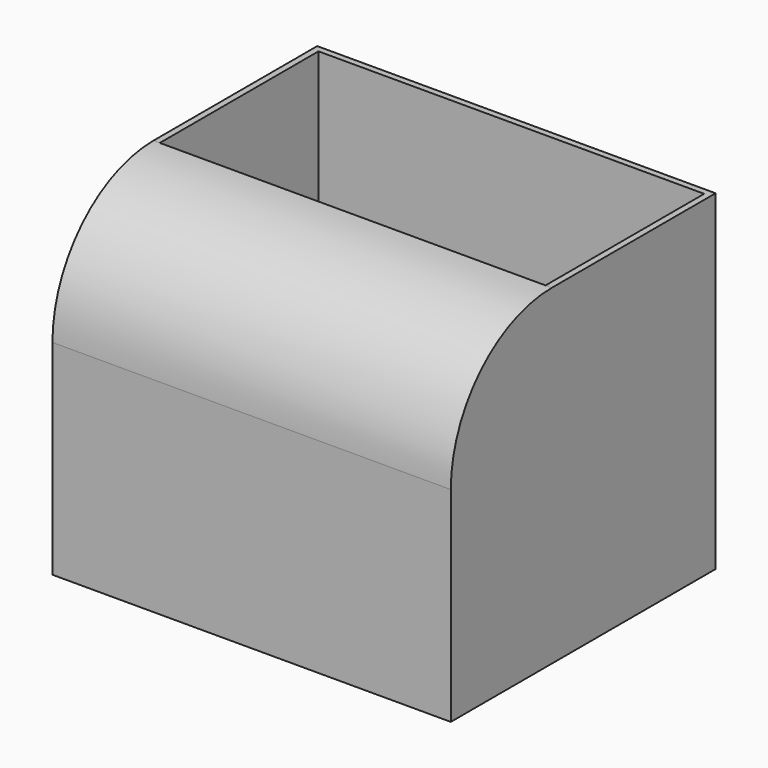
from build123d import *

# Parameters (mm, degrees)
F0_W     = 160.1980030537
F0_H     = 133.0576241016
F1_DEPTH = 133.096
F2_R     = 50.8
F3_T     = -2.54


# Not quite as in the source:
# - a shell that OpenCascade refuses in one call is made with other operations: the cavity is built on its own and cut out


with BuildPart() as f1:
    # F0 (on Front) → F1 (new body)
    with BuildSketch(Plane.XZ):
        with Locations((-80.0990015268, 66.5288120508)):
            Rectangle(F0_W, F0_H)
    extrude(amount=F1_DEPTH)

    # F2
    f2_edges = [f1.edges().sort_by_distance(p)[0] for p in [
        (-80.099002, -133.096, 133.057624),
    ]]
    fillet(f2_edges, radius=F2_R)

    # F3: a shell. OpenCascade refuses it in one call, so the cavity is built on its own and cut out:
    # the body offset inwards by the wall thickness, plus a prism from it out through each open face.
    f3_core = offset(f1.part, amount=F3_T, mode=Mode.PRIVATE)
    f3_exits = [f3_core.faces().sort_by_distance(p)[0] for p in [
        (-80.099002, -42.418, 130.517624),
    ]]
    add(f3_core, mode=Mode.SUBTRACT)
    extrude(f3_exits, amount=-F3_T, mode=Mode.SUBTRACT)


solid = f1.part
